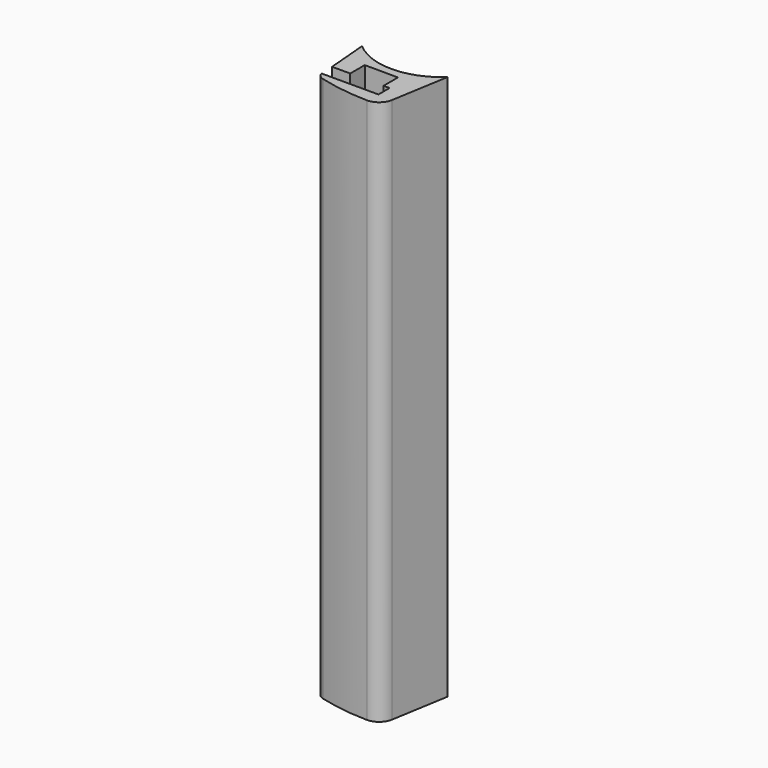
from build123d import *

# Parameters (mm, degrees)
F1_DEPTH    = 180
F2_R        = 5
F3_T1_DEPTH = 191.1494898741


# Not quite as in the source:
# - a fillet or chamfer that OpenCascade refuses, or shapes differently, is made with other operations: its cross-section is extruded or revolved along the edge and cut away or added


with BuildPart() as f1:
    # F0 (on Top) → F1 (new body)
    with BuildSketch(Plane.XY):
        with BuildLine():
            ThreePointArc((14.1226732436, -15.5418821401), (0.1645874713, -20.9993550131), (-13.8773267564, -15.7613388421))
            Line((-13.8773267564, -15.7613388421), (-12.7134246975, -29.6120676683))
            Line((-12.7134246975, -29.6120676683), (-6.7134246975, -29.6071426253))
            Line((-6.7134246975, -29.6071426253), (-6.7134246975, -23.6071426253))
            Line((-6.7134246975, -23.6071426253), (4.2865298223, -23.6563930556))
            Line((4.2865298223, -23.6563930556), (4.2865298223, -29.6071426253))
            Line((4.2865298223, -29.6071426253), (6.2865237583, -29.6120676683))
            Line((6.2865237583, -29.6120676683), (6.2751961593, -34.2120537211))
            Line((6.2751961593, -34.2120537211), (-12.4721404334, -34.2120676683))
            Line((-12.4721404334, -34.2120676683), (-12.4721404334, -35.7862083692))
            ThreePointArc((-12.4721404334, -35.7862083692), (-1.2161640349, -38.1355598231), (10.2751961593, -38.5418821401))
            Line((10.2751961593, -38.5418821401), (14.1226732436, -15.5418821401))
        make_face()
    extrude(amount=F1_DEPTH)

    # F2
    f2_edges = [f1.edges().sort_by_distance(p)[0] for p in [
        (10.275196, -38.541882, 90),
    ]]
    fillet(f2_edges, radius=F2_R)

    # F3: fillet of radius 3 on 1 edges, made by hand

    # F3_s2 → F3_t1 (cut)
    with BuildSketch(Plane.XY.offset(-5.5747449371)):
        with BuildLine():
            ThreePointArc((-10.3257108334, -36.3905964487), (-11.6973730961, -35.5953820953), (-12.4721404334, -34.2120676683))
            Line((-12.4721404334, -34.2120676683), (-12.4721404334, -35.7862083692))
            ThreePointArc((-12.4721404334, -35.7862083692), (-11.4014196416, -36.0972596534), (-10.3257108334, -36.3905964487))
        make_face()
    extrude(amount=F3_T1_DEPTH, mode=Mode.SUBTRACT)


solid = f1.part
